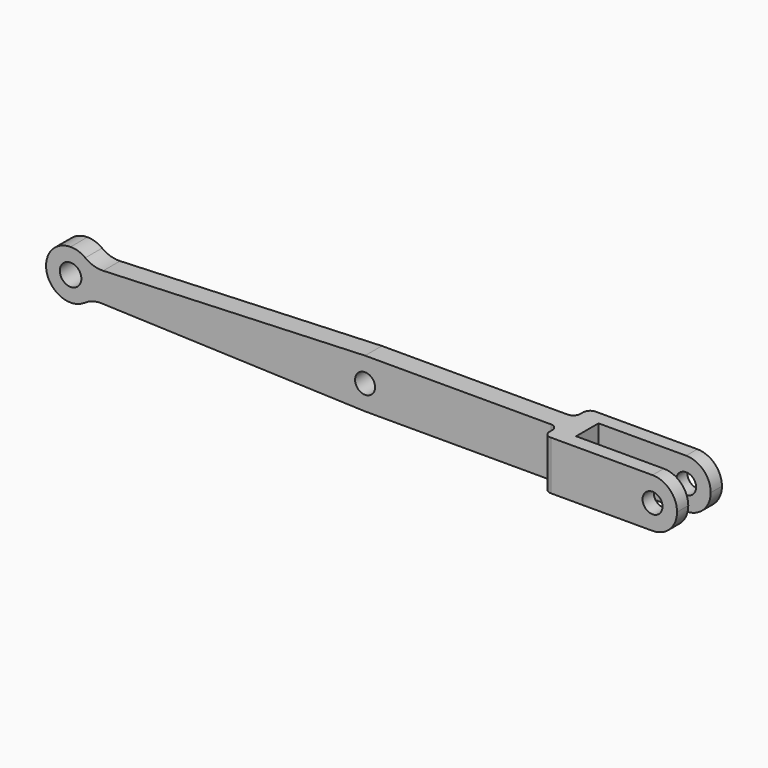
from build123d import *

# Parameters (mm, degrees)
F1_DEPTH = 5.55625
F2_R     = 1.2192
F3_DEPTH = 25.4
F4_R     = 1.1303
F5_DEPTH = 25.4
F6_R     = 2.778115
F7_R     = 2.778115
F8_R     = 1.1303
F9_DEPTH = 25.4


# Not quite as in the source:
# - a fillet or chamfer is up to 0.001 mm smaller than in the source, because OpenCascade refuses the exact size
# - ends of sketch curves that miss each other by under 0.0002 mm in the source are joined


with BuildPart() as f1:
    # F0 (on Top) → F1 (new body)
    with BuildSketch(Plane.XY):
        with BuildLine():
            Line((29.0973595662, 23.0125838354), (-28.0526404338, 23.0125838354))
            Line((-28.0526404338, 23.0125838354), (-28.0526404338, 20.6313338354))
            Line((-28.0526404338, 20.6313338354), (29.0973595662, 20.6313338354))
            ThreePointArc((29.0973595662, 20.6313338354), (29.6586255738, 20.398849843), (29.8911095662, 19.8375838354))
            Line((29.8911095662, 19.8375838354), (29.8911095662, 19.4407088354))
            ThreePointArc((29.8911095662, 19.4407088354), (30.1235935587, 18.8794428278), (30.6848595662, 18.6469588354))
            Line((30.6848595662, 18.6469588354), (44.9723595662, 18.6469588354))
            Line((44.9723595662, 18.6469588354), (44.9723595662, 20.2344588354))
            Line((44.9723595662, 20.2344588354), (32.2723595662, 20.2344588354))
            Line((32.2723595662, 20.2344588354), (32.2723595662, 23.4094588354))
            Line((32.2723595662, 23.4094588354), (44.9723595662, 23.4094588354))
            Line((44.9723595662, 23.4094588354), (44.9723595662, 24.9969588354))
            Line((44.9723595662, 24.9969588354), (30.6848595662, 24.9969588354))
            ThreePointArc((30.6848595662, 24.9969588354), (30.1235935587, 24.764474843), (29.8911095662, 24.2032088354))
            Line((29.8911095662, 24.2032088354), (29.8911095662, 23.8063338354))
            ThreePointArc((29.8911095662, 23.8063338354), (29.6586255738, 23.2450678278), (29.0973595662, 23.0125838354))
        make_face()
    extrude(amount=F1_DEPTH)

    # F2 (on face) → F3 (cut)
    with BuildSketch(Plane.XZ.offset(-20.6313338354)):
        with Locations((-25.2745154338, 2.778125)):
            Circle(F2_R)
    extrude(amount=-F3_DEPTH, mode=Mode.SUBTRACT)

    # F4 (on face) → F5 (cut)
    with BuildSketch(Plane.XZ.offset(-18.6469588354)):
        with Locations((42.1942345662, 2.778125)):
            Circle(F4_R)
    extrude(amount=-F5_DEPTH, mode=Mode.SUBTRACT)

    # F6 (radius 2.778125 in the source; OpenCascade refuses exactly that, so slightly less here)
    f6_edges = [f1.edges().sort_by_distance(p)[0] for p in [
        (44.97236, 19.440709, 5.55625),
        (44.97236, 19.440709, 0),
        (44.97236, 24.203209, 0),
        (44.97236, 24.203209, 5.55625),
    ]]
    fillet(f6_edges, radius=F6_R)

    # F7 (radius 2.778125 in the source; OpenCascade refuses exactly that, so slightly less here)
    f7_edges = [f1.edges().sort_by_distance(p)[0] for p in [
        (-28.05264, 21.821959, 5.55625),
        (-28.05264, 21.821959, 0),
    ]]
    fillet(f7_edges, radius=F7_R)

    # F8 (on face) → F9 (cut)
    with BuildSketch(Plane.XZ.offset(-20.6313338354)):
        with Locations((8.0629845662, 2.778125)):
            Circle(F8_R)
        with BuildLine():
            Line((8.0629845662, 5.55625), (-25.2745254338, 5.55625))
            ThreePointArc((-25.2745254338, 5.55625), (-24.3987826977, 5.4146133255), (-23.612344628, 5.0041453791))
            ThreePointArc((-23.612344628, 5.0041453791), (-22.6534079634, 4.515722008), (-21.5864000573, 4.375682569))
            Line((-21.5864000573, 4.375682569), (8.0629845662, 5.55625))
        make_face()
        with BuildLine():
            ThreePointArc((-23.6851494527, 0.4995521366), (-24.4415033451, 0.1278289079), (-25.2745154338, 0))
            Line((-25.2745154338, 0), (8.0629845662, 0))
            Line((8.0629845662, 0), (-21.7550382738, 1.0684326083))
            ThreePointArc((-21.7550382738, 1.0684326083), (-22.7663528525, 0.9409409702), (-23.6851494527, 0.4995521366))
        make_face()
    extrude(amount=-F9_DEPTH, mode=Mode.SUBTRACT)


solid = f1.part
